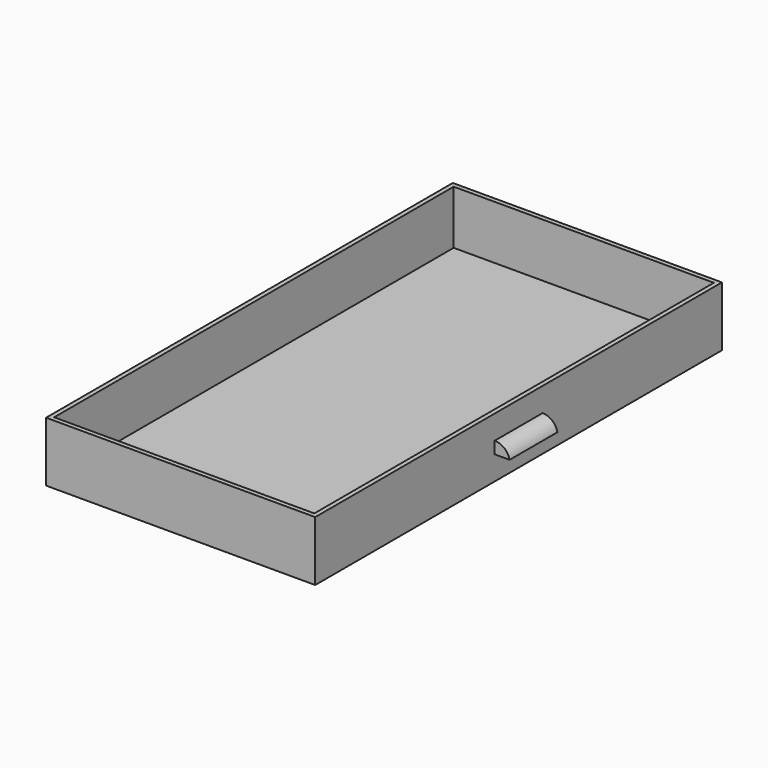
from build123d import *

# Parameters (mm, degrees)
F0_W         = 90
F0_H         = 170
F0_W_2       = 87
F0_H_2       = 167
F1_DEPTH     = 20
F2_DEPTH     = 2
F4_DEPTH     = 5
F5_T         = 1
F5_T3_DEPTH  = 6
F5_T5_DEPTH  = 22
F5_T7_DEPTH  = 89
F5_T9_DEPTH  = 20
F5_T11_DEPTH = 169
F6_T4_DEPTH  = 29.5866302263
F6_T6_DEPTH  = 44.819347292


# Not quite as in the source:
# - a fillet or chamfer that OpenCascade refuses, or shapes differently, is made with other operations: its cross-section is extruded or revolved along the edge and cut away or added
# - a shell that OpenCascade refuses in one call is made with other operations: the cavity is built on its own and cut out


with BuildPart() as f1:
    # F0 (on Top) → F1 (new body)
    with BuildSketch(Plane.XY):
        with Locations((-14.0737314522, 35.681976974)):
            Rectangle(F0_W, F0_H)
        with Locations((-14.0737314522, 35.681976974)):
            Rectangle(F0_W_2, F0_H_2, mode=Mode.SUBTRACT)
    extrude(amount=F1_DEPTH)

    # F0 (on Top) → F2 (join)
    with BuildSketch(Plane.XY):
        with Locations((-14.0737314522, 35.681976974)):
            Rectangle(F0_W_2, F0_H_2)
    extrude(amount=F2_DEPTH)

    # F3 (on face) → F4 (join)
    with BuildSketch(Plane.YZ.offset(30.9262685478)):
        Polygon((45.681976974, 12), (35.681976974, 12), (25.681976974, 12), (25.681976974, 8), (45.681976974, 8), align=None)
    extrude(amount=F4_DEPTH)

    # F5: shell of thickness 1, made by hand


with BuildPart() as f5_core1:
    # F5_t2: copy of F1
    add(f1.part)

    # the walls: a layer under each face that stays
    f5_faces = [f5_core1.faces().sort_by_distance(p)[0] for p in [
        (30.9262685478, -20.9846896927, 16.6666666667),
        (-14.0737314522, -49.318023026, 10),
        (-14.0737314522, 35.681976974, 0),
        (-57.6674814522, 85.0029646283, 20),
        (-14.0737314522, 120.681976974, 10),
        (33.4262685478, 45.681976974, 10),
        (33.4262685478, 25.681976974, 10),
        (33.4262685478, 35.681976974, 12),
        (-59.0737314522, 35.681976974, 10),
        (-14.0737314522, -47.818023026, 11),
        (-57.5737314522, 35.681976974, 11),
        (-14.0737314522, 119.181976974, 11),
        (29.4262685478, 35.681976974, 11),
        (35.9262685478, 35.681976974, 10),
        (-14.0737314522, 35.681976974, 2),
    ]]
    thicken(f5_faces, amount=-F5_T, mode=Mode.SUBTRACT)

    # F5_s4 → F5_t3 (cut)
    with BuildSketch(Plane.XY.offset(7)):
        Polygon((30.9362685478, 45.691976974), (29.9262685478, 45.681976974), (29.9262685478, 44.681976974), (30.9262685478, 44.681976974), align=None)
        Polygon((30.9362685478, 25.671976974), (29.9262685478, 25.681976974), (29.9262685478, 26.681976974), (30.9262685478, 26.681976974), align=None)
    extrude(amount=F5_T3_DEPTH, mode=Mode.SUBTRACT)

    # F5_s6 → F5_t5 (cut)
    with BuildSketch(Plane.XZ.offset(-46.681976974)):
        Polygon((30.9362685478, 12.01), (29.9262685478, 12), (29.9262685478, 11), (30.9262685478, 11), align=None)
    extrude(amount=F5_T5_DEPTH, mode=Mode.SUBTRACT)

    # F5_s8 → F5_t7 (cut)
    with BuildSketch(Plane.YZ.offset(-58.5737314522)):
        Polygon((-47.808023026, 2.01), (-48.818023026, 2), (-48.818023026, 1), (-47.818023026, 1), align=None)
        Polygon((119.171976974, 2.01), (120.181976974, 2), (120.181976974, 1), (119.181976974, 1), align=None)
    extrude(amount=F5_T7_DEPTH, mode=Mode.SUBTRACT)

    # F5_s10 → F5_t9 (cut)
    with BuildSketch(Plane.XY.offset(1)):
        Polygon((-57.5637314522, -47.808023026), (-57.5737314522, -48.818023026), (-58.5737314522, -48.818023026), (-58.5737314522, -47.818023026), align=None)
        Polygon((29.4162685478, -47.808023026), (29.4262685478, -48.818023026), (30.4262685478, -48.818023026), (30.4262685478, -47.818023026), align=None)
        Polygon((-57.5637314522, 119.171976974), (-58.5737314522, 119.181976974), (-58.5737314522, 120.181976974), (-57.5737314522, 120.181976974), align=None)
        Polygon((29.4162685478, 119.171976974), (29.4262685478, 120.181976974), (30.4262685478, 120.181976974), (30.4262685478, 119.181976974), align=None)
    extrude(amount=F5_T9_DEPTH, mode=Mode.SUBTRACT)

    # F5_s12 → F5_t11 (cut)
    with BuildSketch(Plane.XZ.offset(-120.181976974)):
        Polygon((-57.5637314522, 2.01), (-58.5737314522, 2), (-58.5737314522, 1), (-57.5737314522, 1), align=None)
        Polygon((29.4162685478, 2.01), (30.4262685478, 2), (30.4262685478, 1), (29.4262685478, 1), align=None)
    extrude(amount=F5_T11_DEPTH, mode=Mode.SUBTRACT)


with BuildPart() as f1_1:
    add(f1.part)

    # what is left inside the walls is the cavity
    f5_cavity = [f5_core1.part.solids().sort_by_distance(p)[0] for p in [
        (32.676269, 32.681977, 8.01),
    ]]
    add(f5_cavity, mode=Mode.SUBTRACT)

    # F6: fillet of radius 5.08 on 5 edges, made by hand


with BuildPart() as f6_tool2:
    # F6_s3 → F6_t4 (new body)
    with BuildSketch(Plane.XZ.offset(-56.2686072003)):
        with BuildLine():
            ThreePointArc((34.9262685478, 8), (33.0520512056, 10.1845515591), (30.2916164573, 11))
            Line((30.2916164573, 11), (34.9262685478, 11))
            Line((34.9262685478, 11), (34.9262685478, 8))
        make_face()
    extrude(amount=F6_T4_DEPTH)

    split(bisect_by=Plane.XZ.offset(-45.681976974), keep=Keep.TOP)


with BuildPart() as f1_2:
    add(f1_1.part)

    # F6_t1: union F6_tool2
    add(f6_tool2.part)

    # F6_s7 → F6_t6 (cut)
    with BuildSketch(Plane.XZ.offset(-58.09165062)):
        with BuildLine():
            ThreePointArc((35.9262685478, 8), (34.1498745795, 10.8755530587), (30.9623990894, 12))
            Line((30.9623990894, 12), (35.9262685478, 12))
            Line((35.9262685478, 12), (35.9262685478, 8))
        make_face()
    extrude(amount=F6_T6_DEPTH, mode=Mode.SUBTRACT)


solid = f1_2.part
